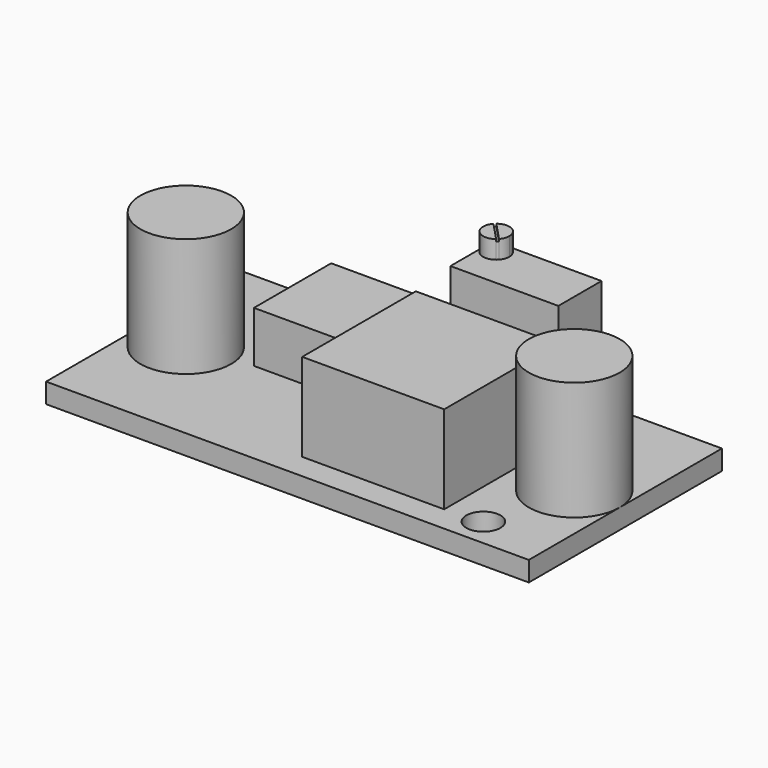
from build123d import *

# Parameters (mm, degrees)
F0_R     = 4
F0_R_2   = 1.5
F0_W     = 12.5
F0_H     = 12.5
F0_W_2   = 9.6
F0_H_2   = 8.5
F0_W_3   = 9.5
F0_H_3   = 4.75
F1_DEPTH = 1.75
F2_DEPTH = 12.2
F3_DEPTH = 6.25
F4_DEPTH = 9.5
F6_DEPTH = 1.6
F7_DEPTH = 1.4


# Not quite as in the source:
# - a feature names something its author has since deleted; it is built from what else it names


with BuildPart() as f1:
    # F0 (on Top) → F1 (new body)
    with BuildSketch(Plane.XY):
        Polygon((-21.25, 10.625), (-21.25, -10.625), (21.25, -10.625), (21.25, -0.625), (21.25, 10.625), align=None)
        with Locations((-16.95, -0.625)):
            Circle(F0_R, mode=Mode.SUBTRACT)
        with Locations((15.25, -8.125)):
            Circle(F0_R_2, mode=Mode.SUBTRACT)
        with Locations((5.75, -2.125)):
            Rectangle(F0_W, F0_H, mode=Mode.SUBTRACT)
        with Locations((17.25, -0.625)):
            Circle(F0_R, mode=Mode.SUBTRACT)
        with Locations((-6.75, 4.375)):
            Rectangle(F0_W_2, F0_H_2, mode=Mode.SUBTRACT)
        with Locations((-14.75, 8.075)):
            Circle(F0_R_2, mode=Mode.SUBTRACT)
        with Locations((7, 6.875)):
            Rectangle(F0_W_3, F0_H_3, mode=Mode.SUBTRACT)
        with Locations((7, 6.875)):
            Rectangle(F0_W_3, F0_H_3)
        with Locations((-6.75, 4.375)):
            Rectangle(F0_W_2, F0_H_2)
        with Locations((17.25, -0.625)):
            Circle(F0_R)
        with Locations((-16.95, -0.625)):
            Circle(F0_R)
    extrude(amount=F1_DEPTH)

    # F0 (on Top) → F2 (join)
    with BuildSketch(Plane.XY):
        with Locations((17.25, -0.625)):
            Circle(F0_R)
        with Locations((7, 6.875)):
            Rectangle(F0_W_3, F0_H_3)
        with Locations((-16.95, -0.625)):
            Circle(F0_R)
    extrude(amount=F2_DEPTH)

    # F0 (on Top) → F3 (join)
    with BuildSketch(Plane.XY):
        with Locations((-6.75, 4.375)):
            Rectangle(F0_W_2, F0_H_2)
    extrude(amount=F3_DEPTH)

    # F0 (on Top) → F4 (join)
    with BuildSketch(Plane.XY):
        with Locations((5.75, -2.125)):
            Rectangle(F0_W, F0_H)
    extrude(amount=F4_DEPTH)

    # F5 (on face) → F6 (join)
    with BuildSketch(Plane.XY.offset(12.2)):
        with BuildLine():
            Line((4.1182401625, 7.1928977493), (2.5462530026, 8.8598879621))
            ThreePointArc((2.5462530026, 8.8598879621), (2.5683356993, 7.3060178406), (4.1182401625, 7.1928977493))
        make_face()
        with BuildLine():
            ThreePointArc((4.2637469974, 7.3301120379), (4.4797229985, 7.6857684317), (4.555, 8.095))
            ThreePointArc((4.555, 8.095), (3.906135617, 9.1300667096), (2.6917598375, 8.9971022507))
            Line((2.6917598375, 8.9971022507), (4.2637469974, 7.3301120379))
        make_face()
    extrude(amount=F6_DEPTH)

    # F5 (on face) → F7 (join)
    with BuildSketch(Plane.XY.offset(12.2)):
        with BuildLine():
            Line((4.2637469974, 7.3301120379), (2.6917598375, 8.9971022507))
            ThreePointArc((2.6917598375, 8.9971022507), (2.6160178406, 8.9316643007), (2.5462530026, 8.8598879621))
            Line((2.5462530026, 8.8598879621), (4.1182401625, 7.1928977493))
            ThreePointArc((4.1182401625, 7.1928977493), (4.1939821594, 7.2583356993), (4.2637469974, 7.3301120379))
        make_face()
    extrude(amount=F7_DEPTH)


solid = f1.part
